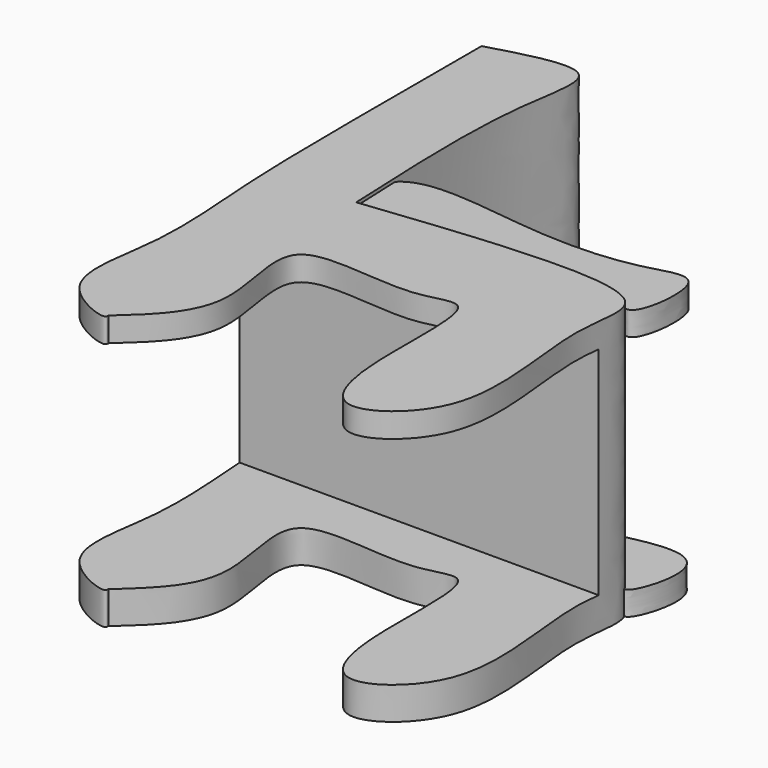
from build123d import *

# Parameters (mm, degrees)
F1_DEPTH      = 80
F2_W          = 74.4883548468
F2_H          = 63.3151000366
F3_DEPTH      = 51.565582156
F3_DEPTH_BACK = 60
F6_DEPTH      = 7
F8_DEPTH      = 7


# Not quite as in the source:
# - a feature of the source that left no trace in its solid (it failed there, or was rolled back) is left out


with BuildPart() as f1:
    # F0 (on Top) → F1 (new body)
    with BuildSketch(Plane.XY):
        with BuildLine():
            add(Edge.make_bspline(
                [(-56.0360439122, 96.469886601), (-56.0360439122, 80.7944474121), (-56.0360439122, 65.1190082232), (-56.0360439122, 49.4435690343)],
                knots=[0, 0, 0, 0, 47.0263175666, 47.0263175666, 47.0263175666, 47.0263175666], degree=3))
            add(Edge.make_bspline(
                [(-56.0360439122, 49.4435690343), (-55.97916634, 35.752272772), (-55.8689178713, 9.2137904003), (-51.9231798075, -25.1424485049), (-60.5293571401, -54.7552799982), (-39.395778527, -63.1034869385), (-39.3452111602, -61.2424431878), (-39.3351055682, -60.8705244958)],
                knots=[0, 0, 0, 0, 0.282533293, 0.5476475473, 0.7796182728, 0.9559580028, 1, 1, 1, 1], degree=3))
            add(Edge.make_bspline(
                [(-39.3351055682, -60.8705244958), (-32.0463849559, -54.3350008389), (-17.4500026501, -41.2469697645), (-34.9648975687, -1.1507715076), (7.4048818648, -12.2877867725), (25.2977205252, -0.5693604358), (20.4554095746, -44.0267518029), (29.1392602503, -67.6741537544), (58.1304151815, -45.8223982246), (45.793229252, -1.3591703757), (57.142981437, 28.1002805174), (4.9446855209, 22.2006747256), (-30.1056392491, 18.2391833514)],
                knots=[0, 0, 0, 0, 0.0955387583, 0.1913257916, 0.2937989011, 0.3599673873, 0.4693871483, 0.5488682741, 0.6374681202, 0.7602344438, 0.8390012458, 1, 1, 1, 1], degree=3))
            add(Edge.make_bspline(
                [(-30.1056392491, 18.2391833514), (-31.1289647813, 40.196685604), (-32.7494951047, 74.9684147438), (-24.1527640362, 105.6269168389), (-45.001540177, 99.6390487686), (-56.0360439122, 96.469886601)],
                knots=[0, 0, 0, 0, 0.4464796453, 0.7070416805, 1, 1, 1, 1], degree=3))
        make_face()
    extrude(amount=F1_DEPTH)

    # F2 (on Right) → F3 (cut, two sides)
    with BuildSketch(Plane.YZ) as f3_sk:
        with Locations((-30.4936701432, 41.2013721652)):
            Rectangle(F2_W, F2_H)
    extrude(amount=F3_DEPTH, mode=Mode.SUBTRACT)
    extrude(f3_sk.sketch, amount=-F3_DEPTH_BACK, mode=Mode.SUBTRACT)


with BuildPart() as f6:
    # F5 (on offset) → F6 (new body)
    with BuildSketch(Plane.XY.offset(79)):
        with BuildLine():
            add(Edge.make_bspline(
                [(-29.7705791891, 18.2560998946), (-33.7327043506, 21.0163114633), (-35.5855507611, 41.7723890529), (8.2143213295, 32.6644025717), (37.9472074704, 33.9946980783), (56.6008398148, 42.0684349474), (53.0015381449, 10.3667837393), (43.2042096436, 23.6911360184), (35.3634214473, 21.8963547001), (22.8134837175, 24.3949285391), (7.1796785413, 21.98173495), (-7.3116275375, 23.0957516435), (-24.9807955753, 14.9193006762), (-29.7705791891, 18.2560998946)],
                knots=[0, 0, 0, 0, 0.084826391, 0.2184272441, 0.3467258803, 0.424330167, 0.5196246269, 0.584833509, 0.6459477341, 0.7236665891, 0.8098448079, 0.8974540073, 1, 1, 1, 1], degree=3))
        make_face()
    extrude(amount=-F6_DEPTH)


with BuildPart() as f8:
    # F7 (on Top) → F8 (new body)
    with BuildSketch(Plane.XY):
        with BuildLine():
            add(Edge.make_bspline(
                [(-29.5314807445, 18.4871889651), (-31.9999912099, 21.2694017994), (-32.4135799943, 38.1531278125), (-23.4440949028, 36.7340414586), (-14.3512568848, 38.5659564346), (-3.6653891037, 34.9265690684), (11.1736303336, 35.6756158748), (21.5387176196, 34.3401530989), (30.7033989329, 36.1042157072), (48.551755128, 40.2824748904), (55.6808399445, 33.366793018), (53.460620713, 20.8596340482), (48.7531355051, 13.3354363986), (41.9907047587, 25.5705691098), (39.9814009229, 21.7790231157), (21.2021126611, 25.6495086732), (19.8213643562, 21.3776182112), (-7.6371083647, 21.8973901153), (-21.6842373728, 20.0408127382), (-27.9685885527, 16.7256818637), (-29.5314807445, 18.4871889651)],
                knots=[0, 0, 0, 0, 0.0700853793, 0.1137668862, 0.1654301574, 0.2226575529, 0.2886202815, 0.3429278512, 0.3961920828, 0.4674754634, 0.5152631752, 0.5758568773, 0.6156957759, 0.6693464703, 0.6960917981, 0.7672116252, 0.7998976243, 0.886193503, 0.9556267257, 1, 1, 1, 1], degree=3))
        make_face()
    extrude(amount=F8_DEPTH)


solid = Compound([f1.part, f6.part, f8.part])
